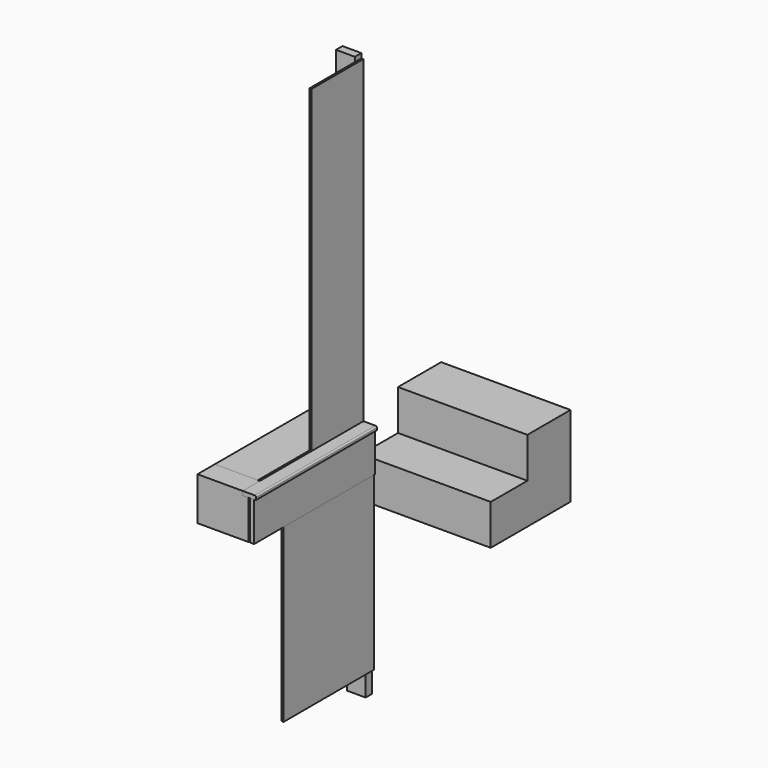
from build123d import *

# Parameters (mm, degrees)
F1_DEPTH      = 38.1
F2_DEPTH      = 304.8
F0_W          = 9.525
F0_H          = 810.9396522522
F3_DEPTH      = 609.6
F4_DEPTH      = 457.2
F0_W_2        = 44.45
F0_H_2        = 38.1
F5_W          = 101.6
F5_H          = 203.2
F6_DEPTH      = 38.1
F6_DEPTH_BACK = 203.2
F7_DEPTH      = 711.2
F8_DEPTH      = 711.2
F9_DEPTH      = 533.4
F11_DEPTH     = 609.6
F12_R         = 6.35
F13_R         = 3.175


with BuildPart() as f1:
    # F0 (on Front) → F1 (new body)
    with BuildSketch(Plane.XZ):
        Polygon((-88.9, 0), (0, 0), (0, 1502.098441124), (0, 1524), (-88.9, 1524), align=None)
    extrude(amount=F1_DEPTH)


with BuildPart() as f1b:
    # F0 (on Front) → F1, piece 2 (new body)
    with BuildSketch(Plane.XZ):
        Polygon((0, -203.2), (-38.1, -203.2), (-38.1, -1117.6), (50.8, -1117.6), (50.8, -1014.1396522522), (50.8, -203.2), (44.45, -203.2), align=None)
    extrude(amount=F1_DEPTH)


with BuildPart() as f2:
    # F0 (on Front) → F2 (new body)
    with BuildSketch(Plane.XZ):
        Polygon((0, 1502.098441124), (0, 0), (0, -15.3818884864), (9.525, -15.3818884864), (9.525, 0), (9.525, 1502.098441124), align=None)
    extrude(amount=F2_DEPTH)


with BuildPart() as f2b:
    # F0 (on Front) → F2, piece 2 (new body)
    with BuildSketch(Plane.XZ):
        with Locations((55.5625, -608.6698261261)):
            Rectangle(F0_W, F0_H)
    extrude(amount=F2_DEPTH)

    # F0 (on Front) → F9 (join)
    with BuildSketch(Plane.XZ):
        with Locations((55.5625, -608.6698261261)):
            Rectangle(F0_W, F0_H)
    extrude(amount=F9_DEPTH)


with BuildPart() as f3:
    # F0 (on Front) → F3 (new body)
    with BuildSketch(Plane.XZ):
        Polygon((0, -15.3818884864), (0, 0), (-88.9, 0), (-203.2, 0), (-203.2, -203.2), (-38.1, -203.2), (0, -203.2), (0, -168.9922213554), (0, -130.8922213554), (0, -63.5), (0, -19.05), align=None)
    extrude(amount=F3_DEPTH)


with BuildPart() as f4:
    # F0 (on Front) → F4 (new body)
    with BuildSketch(Plane.XZ):
        Polygon((9.525, -19.05), (0, -19.05), (0, -63.5), (44.45, -63.5), (44.45, -19.05), align=None)
    extrude(amount=F4_DEPTH)


with BuildPart() as f4b:
    # F0 (on Front) → F4, piece 2 (new body)
    with BuildSketch(Plane.XZ):
        with Locations((22.225, -149.9422213554)):
            Rectangle(F0_W_2, F0_H_2)
    extrude(amount=F4_DEPTH)


with BuildPart() as f6:
    # F5 (on face) → F6 (new body, two sides)
    with BuildSketch(Plane.YZ) as f6_sk:
        with Locations((-660.4, -101.6)):
            Rectangle(F5_W, F5_H)
    extrude(amount=F6_DEPTH)
    extrude(f6_sk.sketch, amount=-F6_DEPTH_BACK)


with BuildPart() as f7:
    # F0 (on Front) → F7 (new body, through all)
    with BuildSketch(Plane.XZ):
        Polygon((44.45, -19.05), (44.45, -63.5), (44.45, -130.8922213554), (44.45, -168.9922213554), (44.45, -203.2), (50.8, -203.2), (60.325, -203.2), (63.5, -203.2), (63.5, -19.05), align=None)
    extrude(amount=F7_DEPTH)


with BuildPart() as f8:
    # F0 (on Front) → F8 (new body, through all)
    with BuildSketch(Plane.XZ):
        Polygon((9.525, 0), (9.525, -15.3818884864), (9.525, -19.05), (44.45, -19.05), (63.5, -19.05), (73.025, -19.05), (73.025, 0), align=None)
    extrude(amount=F8_DEPTH)

    # F12
    f12_edges = [f8.edges().sort_by_distance(p)[0] for p in [
        (73.025, -355.6, 0),
    ]]
    fillet(f12_edges, radius=F12_R)

    # F13
    f13_edges = [f8.edges().sort_by_distance(p)[0] for p in [
        (73.025, -355.6, -19.05),
    ]]
    fillet(f13_edges, radius=F13_R)


with BuildPart() as f11:
    # F10 (on Right) → F11 (new body)
    with BuildSketch(Plane.YZ):
        Polygon((215.9, -139.7), (0, -139.7), (0, -330.2), (469.9, -330.2), (469.9, 50.8), (215.9, 50.8), align=None)
    extrude(amount=F11_DEPTH)


solid = Compound([f1.part, f1b.part, f2.part, f2b.part, f3.part, f4.part, f4b.part, f6.part, f7.part, f8.part, f11.part])
